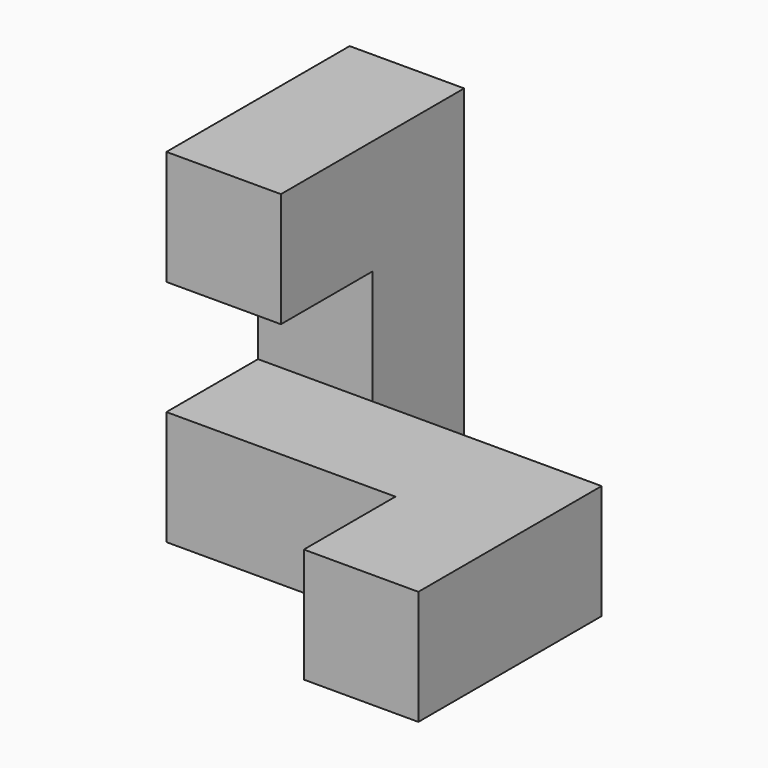
from build123d import *

# Parameters (mm, degrees)
F1_W      = 228.6
F1_H      = 76.2
F2_DEPTH  = 38.1
F3_W      = 76.2
F3_H      = 76.2
F4_DEPTH  = 76.2
F5_W      = 76.2
F5_H      = 76.2
F6_DEPTH  = 76.2
F7_W      = 76.2
F7_H      = 76.2
F8_DEPTH  = 152.4
F9_W      = 76.2
F9_H      = 76.2
F10_DEPTH = 76.2


# Not quite as in the source:
# - a variable given as a bare number and used for a length is read in inches; the dataset says mm whatever the document's units were


with BuildPart() as f2:
    # F1 (on Front) → F2 (new body, symmetric)
    with BuildSketch(Plane.XZ):
        Rectangle(F1_W, F1_H)
    extrude(amount=F2_DEPTH, both=True)

    # F3 (on face) → F4 (join)
    with BuildSketch(Plane.XZ.offset(38.1)):
        with Locations((76.2, 0)):
            Rectangle(F3_W, F3_H)
    extrude(amount=F4_DEPTH)

    # F5 (on face) → F6 (join)
    with BuildSketch(Plane(origin=(0, 38.1, 0), x_dir=(-1, 0, 0), z_dir=(0, 1, 0))):
        with Locations((76.2, 0)):
            Rectangle(F5_W, F5_H)
    extrude(amount=F6_DEPTH)

    # F7 (on face) → F8 (join)
    with BuildSketch(Plane.XY.offset(38.1)):
        with Locations((-76.2, 76.2)):
            Rectangle(F7_W, F7_H)
    extrude(amount=F8_DEPTH)

    # F9 (on face) → F10 (join)
    with BuildSketch(Plane.XZ.offset(-38.1)):
        with Locations((-76.2, 152.4)):
            Rectangle(F9_W, F9_H)
    extrude(amount=F10_DEPTH)


solid = f2.part
